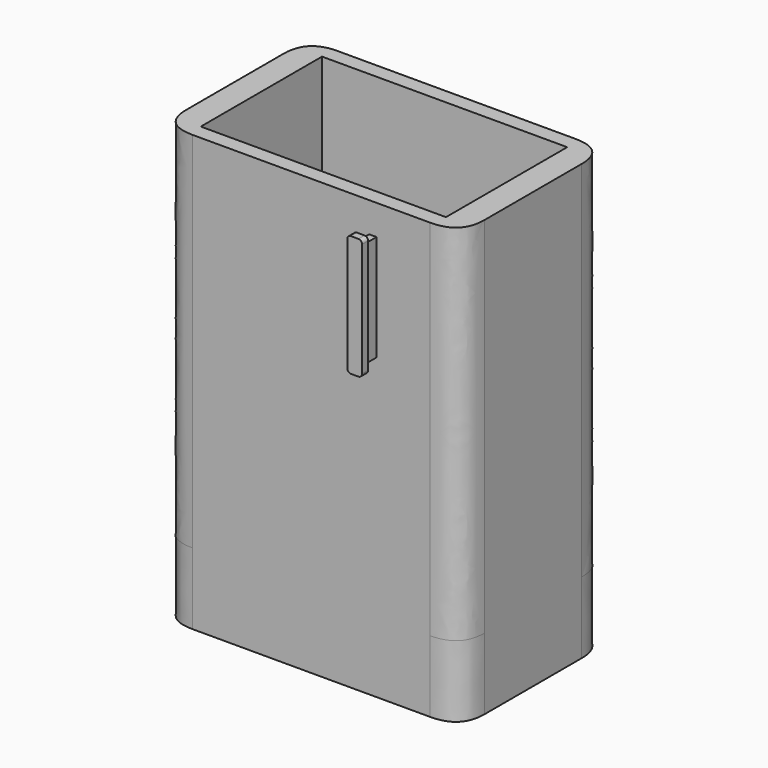
from build123d import *

# Parameters (mm, degrees)
F0_W         = 82.5909674168
F0_H         = 76.3229075819
F1_DEPTH     = 25.4
F2_DEPTH     = 12.7
F3_W         = 71.4602097869
F3_H         = 31.8052172609
F4_DEPTH     = 63.5
F5_W         = 1.5378370881
F5_H         = 22.2577918321
F6_DEPTH     = 3.175
F8_DEPTH     = 1.5875
F9_R         = 0.762
F10_DEPTH    = 20
F11_DEPTH    = 20
F12_T1_DEPTH = 108.0729075819
F13_DEPTH    = 20
F14_DEPTH    = 20
F15_DEPTH    = 5


# Not quite as in the source:
# - a fillet or chamfer that OpenCascade refuses, or shapes differently, is made with other operations: its cross-section is extruded or revolved along the edge and cut away or added
# - a length typed as a fraction of an inch, garbled in the dataset ("3 / 203.2 mm" for 3/8 in), is restored


with BuildPart() as f1:
    # F0 (on Front) → F1 (new body)
    with BuildSketch(Plane.XZ):
        with Locations((8.6646787822, 7.5585497543)):
            Rectangle(F0_W, F0_H)
    extrude(amount=F1_DEPTH)

    # F2 (add): a face of the model
    f2_faces = [f1.faces().sort_by_distance(p)[0] for p in [
        (8.6646787822, -25.4, 7.5585497543),
    ]]
    extrude(f2_faces, amount=F2_DEPTH)

    # F3 (on face) → F4 (cut)
    with BuildSketch(Plane.XY.offset(45.7200035453)):
        with Locations((8.6646787822, -19.05)):
            Rectangle(F3_W, F3_H)
    extrude(amount=-F4_DEPTH, mode=Mode.SUBTRACT)

    # F5 (on face) → F6 (join)
    with BuildSketch(Plane.XZ.offset(38.1)):
        with Locations((11.5634491667, 28.2745240256)):
            Rectangle(F5_W, F5_H)
    extrude(amount=F6_DEPTH)

    # F10 (add): a face of the model
    f10_faces = [f1.faces().sort_by_distance(p)[0] for p in [
        (44.3947836757, -19.05, 13.9700035453),
    ]]
    extrude(f10_faces, amount=F10_DEPTH)

    # F11 (cut): a face of the model
    f11_faces = [f1.faces().sort_by_distance(p)[0] for p in [
        (49.9601624906, -19.05, 7.5585497543),
    ]]
    extrude(f11_faces, amount=-F11_DEPTH, mode=Mode.SUBTRACT)

    # F12: fillet of radius 6.35 on 4 edges, made by hand

    # F12_s2 → F12_t1 (cut)
    with BuildSketch(Plane.XY.offset(-46.4779040366)):
        with BuildLine():
            add(Edge.make_bspline(
                [(29.9601624906, -6.35), (29.9601624906, 0), (23.6101624906, 0)],
                knots=[0, 0, 0, 1, 1, 1], degree=2, weights=[1, 1, 1]))
            Line((23.6101624906, 0), (29.9601624906, 0))
            Line((29.9601624906, 0), (29.9601624906, -6.35))
        make_face()
        with BuildLine():
            add(Edge.make_bspline(
                [(29.9601624906, -31.75), (29.9601624906, -38.1), (23.6101624906, -38.1)],
                knots=[0, 0, 0, 1, 1, 1], degree=2, weights=[1, 1, 1]))
            Line((23.6101624906, -38.1), (29.9601624906, -38.1))
            Line((29.9601624906, -38.1), (29.9601624906, -31.75))
        make_face()
        with BuildLine():
            add(Edge.make_bspline(
                [(-26.2808049262, 0), (-32.6308049262, 0), (-32.6308049262, -6.35)],
                knots=[0, 0, 0, 1, 1, 1], degree=2, weights=[1, 1, 1]))
            Line((-32.6308049262, -6.35), (-32.6308049262, 0))
            Line((-32.6308049262, 0), (-26.2808049262, 0))
        make_face()
        with BuildLine():
            add(Edge.make_bspline(
                [(-32.6308049262, -31.75), (-32.6308049262, -38.1), (-26.2808049262, -38.1)],
                knots=[0, 0, 0, 1, 1, 1], degree=2, weights=[1, 1, 1]))
            Line((-26.2808049262, -38.1), (-32.6308049262, -38.1))
            Line((-32.6308049262, -38.1), (-32.6308049262, -31.75))
        make_face()
    extrude(amount=F12_T1_DEPTH, mode=Mode.SUBTRACT)

    # F13 (add): a face of the model
    f13_faces = [f1.faces().sort_by_distance(p)[0] for p in [
        (-1.3353212302, -19.0499999912, -30.6029040366),
    ]]
    extrude(f13_faces, amount=F13_DEPTH)

    # F14 (cut): a face of the model
    f14_faces = [f1.faces().sort_by_distance(p)[0] for p in [
        (-1.3353212178, -19.05, -17.7799964547),
    ]]
    extrude(f14_faces, amount=-F14_DEPTH, mode=Mode.SUBTRACT)

    # F15 (cut): a face of the model
    f15_faces = [f1.faces().sort_by_distance(p)[0] for p in [
        (-1.3353212302, -19.0499999912, -50.6029040366),
    ]]
    extrude(f15_faces, amount=-F15_DEPTH, mode=Mode.SUBTRACT)


with BuildPart() as f8:
    # F7 (on face) → F8 (new body)
    with BuildSketch(Plane.XZ.offset(41.275)):
        Polygon((10.0171929225, 40.99727422), (10.0171929225, 39.4034199417), (10.0171929225, 17.1456281096), (10.0171929225, 15.5517738312), (13.1097054109, 15.5517738312), (13.1097054109, 17.1456281096), (13.1097054109, 39.4034199417), (13.1097054109, 40.99727422), align=None)
    extrude(amount=F8_DEPTH)

    # F9
    f9_edges = [f8.edges().sort_by_distance(p)[0] for p in [
        (13.109705, -42.06875, 40.997274),
        (10.017193, -42.06875, 40.997274),
        (13.109705, -42.06875, 15.551774),
        (10.017193, -42.06875, 15.551774),
    ]]
    fillet(f9_edges, radius=F9_R)


solid = Compound([f1.part, f8.part])
